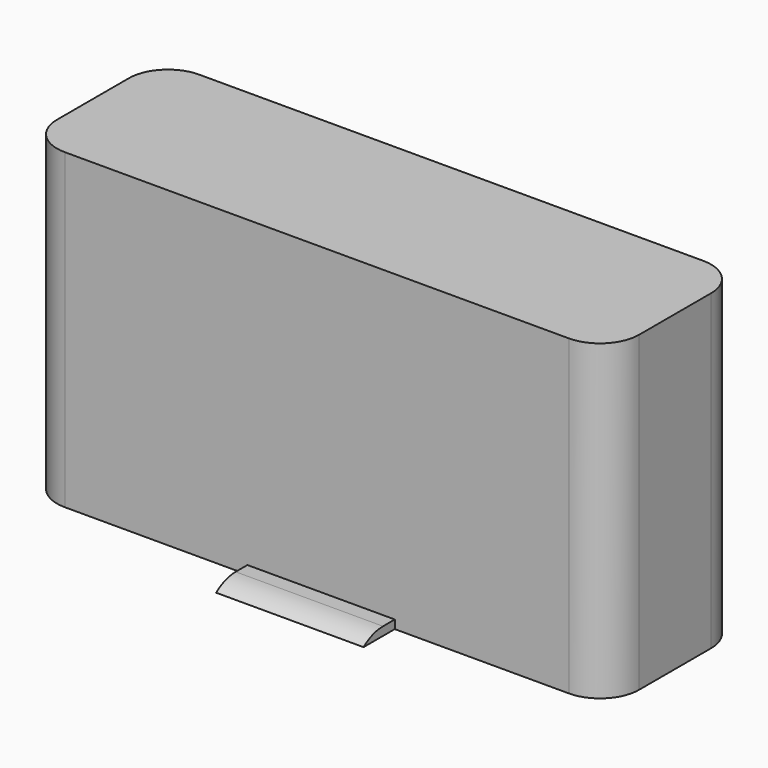
from build123d import *

# Parameters (mm, degrees)
F0_W        = 74.5
F0_H        = 21.5
F0_R        = 10.55
F1_DEPTH    = 40
F2_R        = 5
F7_W        = 18.8593324274
F7_H        = 1.088095014
F8_DEPTH    = 5
F9_T1_DEPTH = 34.4293351412
F10_R       = 3.825
F11_DEPTH   = 25
F12_R       = 3.825
F13_DEPTH   = 25


# Not quite as in the source:
# - a fillet or chamfer that OpenCascade refuses, or shapes differently, is made with other operations: its cross-section is extruded or revolved along the edge and cut away or added


with BuildPart() as f1:
    # F0 (on Top) → F1 (new body)
    with BuildSketch(Plane.XY):
        Rectangle(F0_W, F0_H)
        with Locations((-24.6931102476, 0)):
            Circle(F0_R, mode=Mode.SUBTRACT)
        with BuildLine():
            ThreePointArc((35.3068897524, 0), (24.7568897524, -10.55), (14.2068897524, 0))
            ThreePointArc((14.2068897524, 0), (24.7568897524, 10.55), (35.3068897524, 0))
        make_face(mode=Mode.SUBTRACT)
        with Locations((-24.6931102476, 0)):
            Circle(F0_R)
        with BuildLine():
            ThreePointArc((35.3068897524, 0), (24.7568897524, 10.55), (14.2068897524, 0))
            ThreePointArc((14.2068897524, 0), (24.7568897524, -10.55), (35.3068897524, 0))
        make_face()
    extrude(amount=F1_DEPTH)

    # F2
    f2_edges = [f1.edges().sort_by_distance(p)[0] for p in [
        (-37.25, -10.75, 20),
        (37.25, -10.75, 20),
        (-37.25, 10.75, 20),
        (37.25, 10.75, 20),
    ]]
    fillet(f2_edges, radius=F2_R)

    # F3 (on Front) → F4 (revolve, cut)
    with BuildSketch(Plane.XZ):
        with BuildLine():
            Line((-35.1722761989, 0), (-28.4331102476, 0))
            Line((-28.4331102476, 0), (-28.4331102476, 10.0509282202))
            ThreePointArc((-28.4331102476, 10.0509282202), (-32.7146634372, 5.6369418244), (-35.1722761989, 0))
        make_face()
    revolve(axis=Axis((-24.6931102476, 0, 9.2185929652), (0, 0, 1)), mode=Mode.SUBTRACT)

    # F5 (on Front) → F6 (revolve, cut)
    with BuildSketch(Plane.XZ):
        with BuildLine():
            Line((28.4479595721, 9.307410568), (28.4479595721, 0))
            Line((28.4479595721, 0), (35.168658942, 0))
            ThreePointArc((35.168658942, 0), (32.9055101663, 5.445972629), (28.4479595721, 9.307410568))
        make_face()
    revolve(axis=Axis((24.7338861227, 0, 7.0413234644), (0, 0, 1)), mode=Mode.SUBTRACT)

    # F7 (on face) → F8 (join)
    with BuildSketch(Plane.XZ.offset(10.75)):
        with Locations((0.5516856909, 0.544047507)):
            Rectangle(F7_W, F7_H)
    extrude(amount=F8_DEPTH)

    # F9: fillet of radius 5 on 1 edges, made by hand

    # F9_s2 → F9_t1 (cut)
    with BuildSketch(Plane.YZ.offset(-16.6629818797)):
        with BuildLine():
            ThreePointArc((-12.6359994572, 1.088095014), (-14.2853137193, 0.8082393407), (-15.75, 0))
            Line((-15.75, 0), (-15.75, 1.088095014))
            Line((-15.75, 1.088095014), (-12.6359994572, 1.088095014))
        make_face()
    extrude(amount=F9_T1_DEPTH, mode=Mode.SUBTRACT)

    # F10 (on Top) → F11 (cut)
    with BuildSketch(Plane.XY):
        with Locations((-24.7297555931, 0)):
            Circle(F10_R)
    extrude(amount=F11_DEPTH, mode=Mode.SUBTRACT)

    # F12 (on Top) → F13 (cut)
    with BuildSketch(Plane.XY):
        with Locations((24.8167866624, 0)):
            Circle(F12_R)
    extrude(amount=F13_DEPTH, mode=Mode.SUBTRACT)


solid = f1.part
